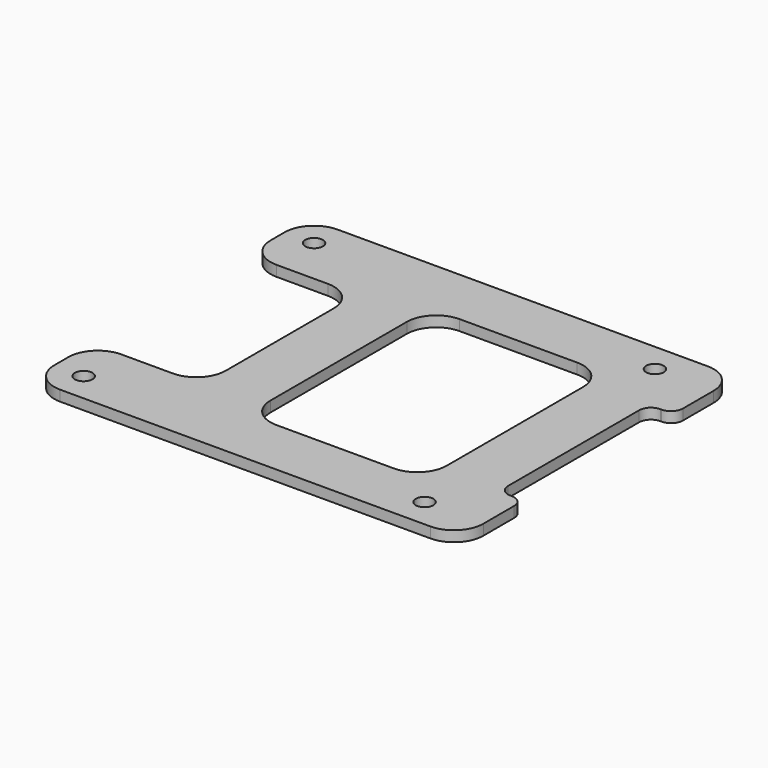
from build123d import *

# Parameters (mm, degrees)
F2_R     = 1.5
F2_W     = 30
F2_H     = 39
F3_DEPTH = 1.8
F5_R     = 5
F6_R     = 2


with BuildPart() as f3:
    # F2 (on Top) → F3 (new body)
    with BuildSketch(Plane.XY):
        Polygon((37.5577017069, 32.9581392366), (-35.4422982931, 32.9581392366), (-35.4422982931, 19.9581392366), (-16.6703661359, 19.9581392366), (-16.6703661359, -13.0418607634), (-35.4422982931, -13.0418607634), (-35.4422982931, -26.0418607634), (37.5577017069, -26.0418607634), (37.5577017069, -12.4774002814), (33.3296338641, -12.4774002814), (33.3296338641, 19.3936787546), (37.5577017069, 19.3936787546), align=None)
        with Locations((-30.4422982931, -21.0418607634)):
            Circle(F2_R, mode=Mode.SUBTRACT)
        with Locations((27.5577017069, -21.0418607634)):
            Circle(F2_R, mode=Mode.SUBTRACT)
        with Locations((8.3296338641, 3.4581392366)):
            Rectangle(F2_W, F2_H, mode=Mode.SUBTRACT)
        with Locations((-30.4422982931, 27.9581392366)):
            Circle(F2_R, mode=Mode.SUBTRACT)
        with Locations((27.5577017069, 27.9581392366)):
            Circle(F2_R, mode=Mode.SUBTRACT)
    extrude(amount=F3_DEPTH)

    # F5
    f5_edges = [f3.edges().sort_by_distance(p)[0] for p in [
        (-6.670366, 22.958139, 0.9),
        (-6.670366, -16.041861, 0.9),
        (23.329634, -16.041861, 0.9),
        (23.329634, 22.958139, 0.9),
        (-35.442298, -26.041861, 0.9),
        (37.557702, 32.958139, 0.9),
        (-35.442298, 32.958139, 0.9),
        (-16.670366, -13.041861, 0.9),
        (-16.670366, 19.958139, 0.9),
        (-35.442298, 19.958139, 0.9),
        (-35.442298, -13.041861, 0.9),
        (37.557702, -26.041861, 0.9),
    ]]
    fillet(f5_edges, radius=F5_R)

    # F6
    f6_edges = [f3.edges().sort_by_distance(p)[0] for p in [
        (37.557702, 19.393679, 0.9),
        (37.557702, -12.4774, 0.9),
        (33.329634, 19.393679, 0.9),
        (33.329634, -12.4774, 0.9),
    ]]
    fillet(f6_edges, radius=F6_R)


solid = f3.part
